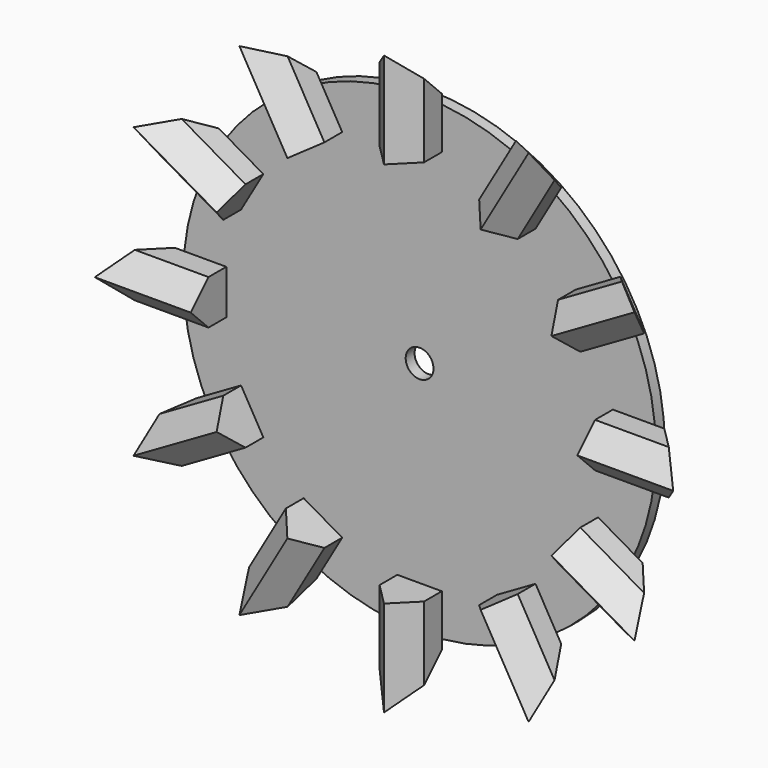
from build123d import *

# Parameters (mm, degrees)
F1_W     = 10.16
F1_H     = 21.9076174819
F2_DEPTH = 10.16
F3_SIZE  = 5.07999
F4_SIZE  = 10.15999
F5_COUNT = 12
F0_R     = 53.975
F6_DEPTH = 2.54
F7_R     = 3.175
F8_DEPTH = 25.4


# Not quite as in the source:
# - a fillet or chamfer is up to 0.001 mm smaller than in the source, because OpenCascade refuses the exact size


with BuildPart() as f2:
    # F1 (on face) → F2 (new body)
    with BuildSketch(Plane.XZ):
        with Locations((0, 55.101165548)):
            Rectangle(F1_W, F1_H)
    extrude(amount=F2_DEPTH)

    # F3 (size 5.08 in the source; OpenCascade refuses exactly that, so slightly less here)
    f3_edges = [f2.edges().sort_by_distance(p)[0] for p in [
        (-5.08, -10.16, 55.101166),
        (5.08, -10.16, 55.101166),
    ]]
    chamfer(f3_edges, length=F3_SIZE)

    # F4 (size 10.16 in the source; OpenCascade refuses exactly that, so slightly less here)
    f4_edges = [f2.edges().sort_by_distance(p)[0] for p in [
        (0, 0, 66.054974),
    ]]
    chamfer(f4_edges, length=F4_SIZE)


with BuildPart() as f5_1:
    # F5: instance of F2
    add(f2.part.rotate(Axis((0, 0, 0), (0, -1, 0)), 1 * 360 / F5_COUNT))


with BuildPart() as f5_2:
    # F5: instance of F2
    add(f2.part.rotate(Axis((0, 0, 0), (0, -1, 0)), 2 * 360 / F5_COUNT))


with BuildPart() as f5_3:
    # F5: instance of F2
    add(f2.part.rotate(Axis((0, 0, 0), (0, -1, 0)), 3 * 360 / F5_COUNT))


with BuildPart() as f5_4:
    # F5: instance of F2
    add(f2.part.rotate(Axis((0, 0, 0), (0, -1, 0)), 4 * 360 / F5_COUNT))


with BuildPart() as f5_5:
    # F5: instance of F2
    add(f2.part.rotate(Axis((0, 0, 0), (0, -1, 0)), 5 * 360 / F5_COUNT))


with BuildPart() as f5_6:
    # F5: instance of F2
    add(f2.part.rotate(Axis((0, 0, 0), (0, -1, 0)), 6 * 360 / F5_COUNT))


with BuildPart() as f5_7:
    # F5: instance of F2
    add(f2.part.rotate(Axis((0, 0, 0), (0, -1, 0)), 7 * 360 / F5_COUNT))


with BuildPart() as f5_8:
    # F5: instance of F2
    add(f2.part.rotate(Axis((0, 0, 0), (0, -1, 0)), 8 * 360 / F5_COUNT))


with BuildPart() as f5_9:
    # F5: instance of F2
    add(f2.part.rotate(Axis((0, 0, 0), (0, -1, 0)), 9 * 360 / F5_COUNT))


with BuildPart() as f5_10:
    # F5: instance of F2
    add(f2.part.rotate(Axis((0, 0, 0), (0, -1, 0)), 10 * 360 / F5_COUNT))


with BuildPart() as f5_11:
    # F5: instance of F2
    add(f2.part.rotate(Axis((0, 0, 0), (0, -1, 0)), 11 * 360 / F5_COUNT))


with BuildPart() as f6:
    # F0 (on Front) → F6 (new body)
    with BuildSketch(Plane.XZ):
        Circle(F0_R)
    extrude(amount=-F6_DEPTH)

    # F7 (on face) → F8 (cut)
    with BuildSketch(Plane.XZ):
        Circle(F7_R)
    extrude(amount=-F8_DEPTH, mode=Mode.SUBTRACT)


solid = Compound([f2.part, f5_1.part, f5_2.part, f5_3.part, f5_4.part, f5_5.part, f5_6.part, f5_7.part, f5_8.part, f5_9.part, f5_10.part, f5_11.part, f6.part])
